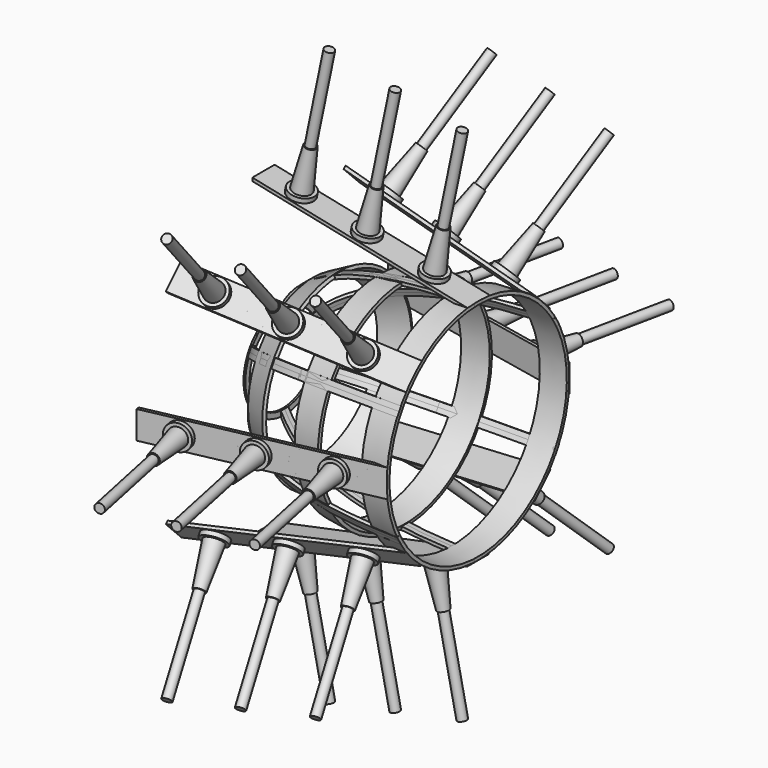
from build123d import *

# Parameters (mm, degrees)
F1_DEPTH  = 0.254
F2_W      = 0.1021561111
F2_H      = 0.292079756
F4_COUNT  = 6
F8_DEPTH  = 0.762
F9_COUNT  = 8
F12_R     = 0.6986880185
F13_DEPTH = 0.254
F14_R     = 0.5166743248
F15_DEPTH = 2.54
F17_R     = 0.254
F18_DEPTH = 7.62
F19_COUNT = 8


# Not quite as in the source:
# - a fillet or chamfer that OpenCascade refuses, or shapes differently, is made with other operations: its cross-section is extruded or revolved along the edge and cut away or added


with BuildPart() as f1:
    # F0 (on Front) → F1 (new body, symmetric)
    with BuildSketch(Plane.XZ):
        with BuildLine():
            add(Edge.make_bspline(
                [(0, 2.6890891604), (1.3812376419, 5.5280539673), (5.9911650605, 6.1729203444), (10.5971740559, 6.2402983312)],
                knots=[0, 0, 0, 0, 11.1763672338, 11.1763672338, 11.1763672338, 11.1763672338], degree=3))
            Line((0, 2.6890891604), (0, 2.384288935))
            add(Edge.make_bspline(
                [(0, 2.384288935), (1.4862640528, 5.3780893795), (5.9911650605, 5.9968786663), (10.5971740559, 6.0642566532)],
                knots=[0, 0, 0, 0, 11.2179436787, 11.2179436787, 11.2179436787, 11.2179436787], degree=3))
            Line((10.5971740559, 6.0642566532), (10.5971740559, 6.2402983312))
        make_face()
    extrude(amount=F1_DEPTH, both=True)


with BuildPart() as f1b:
    # F0 (on Front) → F1, piece 2 (new body, symmetric)
    with BuildSketch(Plane.XZ):
        with BuildLine():
            Line((0, -2.384298), (0, -2.689098))
            add(Edge.make_bspline(
                [(0, -2.689098), (1.3812376419, -5.5280628069), (5.9911650605, -6.1729136912), (10.5971740559, -6.2402916781)],
                knots=[0, 0, 0, 0, 11.1763623111, 11.1763623111, 11.1763623111, 11.1763623111], degree=3))
            Line((10.5971740559, -6.2402916781), (10.5971740559, -6.06425))
            add(Edge.make_bspline(
                [(0, -2.384298), (1.4862640528, -5.3780984445), (5.9911650605, -5.9968720131), (10.5971740559, -6.06425)],
                knots=[0, 0, 0, 0, 11.2179385224, 11.2179385224, 11.2179385224, 11.2179385224], degree=3))
        make_face()
    extrude(amount=F1_DEPTH, both=True)


with BuildPart() as f3:
    # F2 (on Front) → F3 (revolve)
    with BuildSketch(Plane.XZ):
        with Locations((-0.0510780555, 2.5376320118)):
            Rectangle(F2_W, F2_H)
    revolve(axis=Axis((2.0852676389, 0, 0), (1, 0, 0)))


with BuildPart() as f4_1:
    # F4: instance of F1
    add(f1.part.rotate(Axis((0, 0, 0), (1, 0, 0)), 1 * 360 / F4_COUNT))


with BuildPart() as f4_2:
    # F4: instance of F1
    add(f1.part.rotate(Axis((0, 0, 0), (1, 0, 0)), 2 * 360 / F4_COUNT))


with BuildPart() as f4_3:
    # F4: instance of F1
    add(f1.part.rotate(Axis((0, 0, 0), (1, 0, 0)), 3 * 360 / F4_COUNT))


with BuildPart() as f4_4:
    # F4: instance of F1
    add(f1.part.rotate(Axis((0, 0, 0), (1, 0, 0)), 4 * 360 / F4_COUNT))


with BuildPart() as f4_5:
    # F4: instance of F1
    add(f1.part.rotate(Axis((0, 0, 0), (1, 0, 0)), 5 * 360 / F4_COUNT))


with BuildPart() as f4_6:
    # F4: instance of F1b
    add(f1b.part.rotate(Axis((0, 0, 0), (1, 0, 0)), 1 * 360 / F4_COUNT))


with BuildPart() as f4_7:
    # F4: instance of F1b
    add(f1b.part.rotate(Axis((0, 0, 0), (1, 0, 0)), 2 * 360 / F4_COUNT))


with BuildPart() as f4_8:
    # F4: instance of F1b
    add(f1b.part.rotate(Axis((0, 0, 0), (1, 0, 0)), 3 * 360 / F4_COUNT))


with BuildPart() as f4_9:
    # F4: instance of F1b
    add(f1b.part.rotate(Axis((0, 0, 0), (1, 0, 0)), 4 * 360 / F4_COUNT))


with BuildPart() as f4_10:
    # F4: instance of F1b
    add(f1b.part.rotate(Axis((0, 0, 0), (1, 0, 0)), 5 * 360 / F4_COUNT))


with BuildPart() as f6:
    # F5 (on Front) → F6 (revolve)
    with BuildSketch(Plane.XZ):
        Polygon((10.5980772543, 6.0692786596), (10.5899824346, 6.2479329355), (9.1621999513, 6.1832401556), (9.170294771, 6.0045858798), align=None)
    revolve(axis=Axis((5.5151926354, 0, 0), (1, 0, 0)))


with BuildPart() as f6b:
    # F5 (on Front) → F6, piece 2 (revolve)
    with BuildSketch(Plane.XZ):
        Polygon((6.6126598978, 5.7789162553), (6.5890251352, 5.9561851877), (5.1684811167, 5.7667880941), (5.1921158792, 5.5895191617), align=None)
    revolve(axis=Axis((5.5151926354, 0, 0), (1, 0, 0)))


with BuildPart() as f6c:
    # F5 (on Front) → F6, piece 3 (revolve)
    with BuildSketch(Plane.XZ):
        Polygon((2.9757019956, 4.9828256978), (2.8912533694, 5.1444001993), (1.55780637, 4.4474599882), (1.6422549961, 4.2858854868), align=None)
    revolve(axis=Axis((5.5151926354, 0, 0), (1, 0, 0)))


with BuildPart() as f8:
    # F7 (on Front) → F8 (new body, symmetric)
    with BuildSketch(Plane.XZ):
        Polygon((10.5968834832, 6.2437811866), (-1.155209272, 8.693730136), (-1.155209272, 8.5157673517), (9.8840836436, 6.2144151889), align=None)
    extrude(amount=F8_DEPTH, both=True)


with BuildPart() as f9_1:
    # F9: instance of F8
    add(f8.part.rotate(Axis((9.1621999513, 0, 0), (1, 0, 0)), 1 * 360 / F9_COUNT))


with BuildPart() as f9_2:
    # F9: instance of F8
    add(f8.part.rotate(Axis((9.1621999513, 0, 0), (1, 0, 0)), 2 * 360 / F9_COUNT))


with BuildPart() as f9_3:
    # F9: instance of F8
    add(f8.part.rotate(Axis((9.1621999513, 0, 0), (1, 0, 0)), 3 * 360 / F9_COUNT))


with BuildPart() as f9_4:
    # F9: instance of F8
    add(f8.part.rotate(Axis((9.1621999513, 0, 0), (1, 0, 0)), 4 * 360 / F9_COUNT))


with BuildPart() as f9_5:
    # F9: instance of F8
    add(f8.part.rotate(Axis((9.1621999513, 0, 0), (1, 0, 0)), 5 * 360 / F9_COUNT))


with BuildPart() as f9_6:
    # F9: instance of F8
    add(f8.part.rotate(Axis((9.1621999513, 0, 0), (1, 0, 0)), 6 * 360 / F9_COUNT))


with BuildPart() as f9_7:
    # F9: instance of F8
    add(f8.part.rotate(Axis((9.1621999513, 0, 0), (1, 0, 0)), 7 * 360 / F9_COUNT))


with BuildPart() as f8_1:
    add(f8.part)

    # F12 (on offset) → F13 (join)
    with BuildSketch(Plane(origin=(1.6887767476, 0, 8.1008467487), x_dir=(0.9789538613, 0, -0.2040816929), z_dir=(0.2040816929, 0, 0.9789538613))):
        with Locations((-0.8082210291, 0)):
            Circle(F12_R)
        with Locations((2.8751550079, 0)):
            Circle(F12_R)
        with Locations((6.625440989, 0)):
            Circle(F12_R)
    extrude(amount=F13_DEPTH)

    # F14 (on offset) → F15 (join)
    with BuildSketch(Plane(origin=(1.6887767476, 0, 8.1008467487), x_dir=(0.9789538613, 0, -0.2040816929), z_dir=(0.2040816929, 0, 0.9789538613))):
        with Locations((-0.8082210291, 0)):
            Circle(F14_R)
        with Locations((2.8751550079, 0)):
            Circle(F14_R)
        with Locations((6.625440989, 0)):
            Circle(F14_R)
    extrude(amount=F15_DEPTH)

    # F16: chamfer of 0.2032 x 2.3225866279 on 3 edges, made by hand


with BuildPart() as f16_tool2:
    # F16_s3 → F16_t4 (revolve)
    with BuildSketch(Plane.XZ):
        Polygon((1.4477360647, 8.3731837537), (1.7228100509, 10.6883583014), (1.9217334755, 10.6468889015), align=None)
    revolve(axis=Axis((1.4159331502, 0, 10.7523326723), (0.2040816929, 0, 0.9789538613)))

    split(bisect_by=Plane(origin=(1.7406134976, 0, 8.3495010295), x_dir=(0, 1, 0), z_dir=(0.2040816929, 0, 0.9789538613)), keep=Keep.TOP)


with BuildPart() as f8_2:
    add(f8_1.part)

    # F16_t1: cut F16_tool2
    add(f16_tool2.part, mode=Mode.SUBTRACT)


with BuildPart() as f16_tool7:
    # F16_s8 → F16_t9 (revolve)
    with BuildSketch(Plane.XZ):
        Polygon((5.0535912589, 7.6214741367), (5.3286652451, 9.9366486844), (5.5275886697, 9.8951792844), align=None)
    revolve(axis=Axis((5.0217883444, 0, 10.0006230553), (0.2040816929, 0, 0.9789538613)))

    split(bisect_by=Plane(origin=(1.7406134976, 0, 8.3495010295), x_dir=(0, 1, 0), z_dir=(0.2040816929, 0, 0.9789538613)), keep=Keep.TOP)


with BuildPart() as f8_3:
    add(f8_2.part)

    # F16_t6: cut F16_tool7
    add(f16_tool7.part, mode=Mode.SUBTRACT)


with BuildPart() as f16_tool12:
    # F16_s13 → F16_t14 (revolve)
    with BuildSketch(Plane.XZ):
        Polygon((8.7249482012, 6.856109425), (9.0000221874, 9.1712839727), (9.198945612, 9.1298145727), align=None)
    revolve(axis=Axis((8.6931452867, 0, 9.2352583436), (0.2040816929, 0, 0.9789538613)))

    split(bisect_by=Plane(origin=(1.7406134976, 0, 8.3495010295), x_dir=(0, 1, 0), z_dir=(0.2040816929, 0, 0.9789538613)), keep=Keep.TOP)


with BuildPart() as f8_4:
    add(f8_3.part)

    # F16_t11: cut F16_tool12
    add(f16_tool12.part, mode=Mode.SUBTRACT)

    # F17 (on offset) → F18 (join)
    with BuildSketch(Plane(origin=(1.6887767476, 0, 8.1008467487), x_dir=(0.9789538613, 0, -0.2040816929), z_dir=(0.2040816929, 0, 0.9789538613))):
        with Locations((-0.8082210291, 0)):
            Circle(F17_R)
        with Locations((2.8751550079, 0)):
            Circle(F17_R)
        with Locations((6.625440989, 0)):
            Circle(F17_R)
    extrude(amount=F18_DEPTH)


with BuildPart() as f19_1:
    # F19: instance of F8
    add(f8_4.part.rotate(Axis((10.5899824346, 0, 0), (-1, 0, 0)), 1 * 360 / F19_COUNT))


with BuildPart() as f19_2:
    # F19: instance of F8
    add(f8_4.part.rotate(Axis((10.5899824346, 0, 0), (-1, 0, 0)), 2 * 360 / F19_COUNT))


with BuildPart() as f19_3:
    # F19: instance of F8
    add(f8_4.part.rotate(Axis((10.5899824346, 0, 0), (-1, 0, 0)), 3 * 360 / F19_COUNT))


with BuildPart() as f19_4:
    # F19: instance of F8
    add(f8_4.part.rotate(Axis((10.5899824346, 0, 0), (-1, 0, 0)), 4 * 360 / F19_COUNT))


with BuildPart() as f19_5:
    # F19: instance of F8
    add(f8_4.part.rotate(Axis((10.5899824346, 0, 0), (-1, 0, 0)), 5 * 360 / F19_COUNT))


with BuildPart() as f19_6:
    # F19: instance of F8
    add(f8_4.part.rotate(Axis((10.5899824346, 0, 0), (-1, 0, 0)), 6 * 360 / F19_COUNT))


with BuildPart() as f19_7:
    # F19: instance of F8
    add(f8_4.part.rotate(Axis((10.5899824346, 0, 0), (-1, 0, 0)), 7 * 360 / F19_COUNT))


solid = Compound([f1.part, f1b.part, f3.part, f4_1.part, f4_2.part, f4_3.part, f4_4.part, f4_5.part, f4_6.part, f4_7.part, f4_8.part, f4_9.part, f4_10.part, f6.part, f6b.part, f6c.part, f9_1.part, f9_2.part, f9_3.part, f9_4.part, f9_5.part, f9_6.part, f9_7.part, f8_4.part, f19_1.part, f19_2.part, f19_3.part, f19_4.part, f19_5.part, f19_6.part, f19_7.part])
